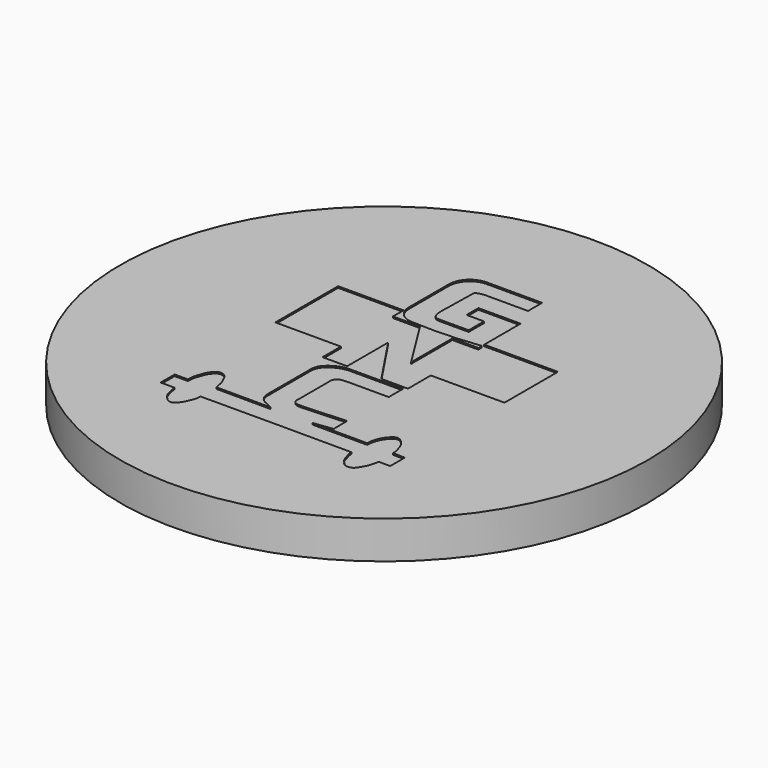
from build123d import *

# Parameters (mm, degrees)
F0_R     = 44.45
F1_DEPTH = 6.35
F3_DEPTH = 0.254


# Not quite as in the source:
# - ends of sketch curves that miss each other by under 0.0002 mm in the source are joined


with BuildPart() as f1:
    # F0 (on Top) → F1 (new body)
    with BuildSketch(Plane.XY):
        Circle(F0_R)
    extrude(amount=F1_DEPTH)

    # F2 (on face) → F3 (cut)
    with BuildSketch(Plane.XY.offset(6.35)):
        with BuildLine():
            Line((5.6039993651, 23.2917912652), (5.6039993651, 26.2641511811))
            Line((5.6039993651, 26.2641511811), (-3.5374157604, 26.2641511811))
            ThreePointArc((-3.5374157604, 26.2641511811), (-6.1724008767, 25.2877017598), (-7.2804156008, 22.7052797559))
            Line((-7.2804156008, 22.7052797559), (-7.2804156008, 14.3152289093))
            ThreePointArc((-7.2804156008, 14.3152289093), (-6.4557803762, 12.2478717336), (-4.4346582144, 11.3156409934))
            ThreePointArc((-4.4346582144, 11.3156409934), (1.3092272973, 11.2673019991), (7.0349466987, 11.7263169959))
            Line((7.0349466987, 11.7263169959), (7.0961336605, 12.2146336362))
            Line((7.0961336605, 12.2146336362), (7.0961336605, 19.8627323627))
            Line((7.0961336605, 19.8627323627), (0, 19.8627323627))
            Line((0, 19.8627323627), (0, 17.358450219))
            Line((0, 17.358450219), (2.9400843196, 17.3616167158))
            Line((2.9400843196, 17.3616167158), (2.9400843196, 14.1317071393))
            Line((2.9400843196, 14.1317071393), (0, 14.1317071393))
            Line((0, 14.1317071393), (-2.2346060723, 14.1317071393))
            ThreePointArc((-2.2346060723, 14.1317071393), (-2.7898678793, 14.3800667532), (-3.1146267429, 14.8943914101))
            ThreePointArc((-3.1146267429, 14.8943914101), (-3.2355914853, 15.5005322545), (-3.2674165577, 16.1178055789))
            Line((-3.2674165577, 16.1178055789), (-3.1592417437, 21.2145812126))
            ThreePointArc((-3.1592417437, 21.2145812126), (-3.1837866635, 21.575252567), (-3.1439608429, 21.9345577061))
            ThreePointArc((-3.1439608429, 21.9345577061), (-3.117530452, 22.198564373), (-3.1439608429, 22.4625710398))
            ThreePointArc((-3.1439608429, 22.4625710398), (-3.0817290753, 22.8241742068), (-2.7919525746, 23.0492502451))
            ThreePointArc((-2.7919525746, 23.0492502451), (-2.1422008965, 23.2306538656), (-1.4703774561, 23.2917912652))
            Line((-1.4703774561, 23.2917912652), (5.6039993651, 23.2917912652))
        make_face()
        with BuildLine():
            Line((-3.1592417437, 21.2145812126), (-3.1439608429, 21.9345577061))
            ThreePointArc((-3.1439608429, 21.9345577061), (-3.1837866635, 21.575252567), (-3.1592417437, 21.2145812126))
        make_face()
        Polygon((7.0961336605, 12.2146336362), (7.0349466987, 11.7263169959), (7.0961336605, 10.9925279394), (7.0961336605, 0.9659290663), (19.5016358048, 0.9659290663), (19.5016358048, 12.2146336362), align=None)
        Polygon((7.0961336605, 0.9659290663), (7.0961336605, 10.9925279394), (2.7143813204, 10.9925279394), (2.7143813204, 2.2997791572), (-2.7398910557, 10.9925279394), (-7.300500758, 10.9925279394), (-7.2804156008, 0), (-7.2804156008, -3.8537723012), (-6.2781353481, -3.8537723012), (-3.1410043308, -3.8537723012), (-3.1410043308, 4.7863919603), (2.6191033489, -3.8537723012), (7.0961336605, -3.8537723012), align=None)
        Polygon((-7.2804156008, 0), (-7.300500758, 10.9925279394), (-7.2804156008, 13.206558302), (-18.3086954057, 13.206558302), (-18.3086954057, 0), align=None)
        with BuildLine():
            Line((0, -7.2983574902), (6.6179535352, -7.2983574902))
            Line((6.6179535352, -7.2983574902), (6.6179535352, -4.2878086955))
            Line((6.6179535352, -4.2878086955), (-2.2489061664, -4.2878086955))
            ThreePointArc((-2.2489061664, -4.2878086955), (-4.0568875501, -4.6442817118), (-5.5942512015, -5.6603440615))
            ThreePointArc((-5.5942512015, -5.6603440615), (-6.1507192567, -6.4794007942), (-6.3533238135, -7.4486592847))
            Line((-6.3533238135, -7.4486592847), (-6.3533238135, -16.6105034737))
            ThreePointArc((-6.3533238135, -16.6105034737), (-5.8759308245, -17.9913268961), (-4.6476325952, -18.782440573))
            Line((-4.6476325952, -18.782440573), (-3.7075637703, -19.2863568686))
            Line((-3.7075637703, -19.2863568686), (3.3881619917, -19.303988614))
            Line((3.3881619917, -19.303988614), (6.6293859856, -18.9052186906))
            Line((6.6293859856, -18.9052186906), (6.593650474, -16.0276701207))
            Line((6.593650474, -16.0276701207), (0, -16.3928680122))
            ThreePointArc((0, -16.3928680122), (-0.7145080017, -16.4126398372), (-1.4290160034, -16.3928680122))
            ThreePointArc((-1.4290160034, -16.3928680122), (-2.080113152, -16.0523673946), (-2.251843689, -15.3379607946))
            Line((-2.251843689, -15.3379607946), (-2.251843689, -8.4599647671))
            ThreePointArc((-2.251843689, -8.4599647671), (-2.0899663646, -7.8730095416), (-1.6501033679, -7.4520092458))
            ThreePointArc((-1.6501033679, -7.4520092458), (-0.8286208401, -7.3368533365), (0, -7.2983574902))
        make_face()
        with BuildLine():
            Line((3.3881619917, -19.303988614), (-3.7075637703, -19.2863568686))
            Line((-3.7075637703, -19.2863568686), (-12.6563319936, -19.2641206086))
            Line((-12.6563319936, -19.2641206086), (-12.8377182409, -19.2641206086))
            Line((-12.8377182409, -19.2641206086), (-12.9873463884, -18.6591409147))
            ThreePointArc((-12.9873463884, -18.6591409147), (-13.1098010784, -17.8878071535), (-13.4031539783, -17.1640012413))
            ThreePointArc((-13.4031539783, -17.1640012413), (-13.5725884432, -16.8395453931), (-13.7304924428, -16.5093243122))
            ThreePointArc((-13.7304924428, -16.5093243122), (-14.0521811274, -16.0543913958), (-14.5178735256, -15.7484859228))
            ThreePointArc((-14.5178735256, -15.7484859228), (-15.086809482, -15.6747136098), (-15.6148988754, -15.8988833427))
            ThreePointArc((-15.6148988754, -15.8988833427), (-16.1466107031, -16.4449553577), (-16.5172908455, -17.1109195799))
            ThreePointArc((-16.5172908455, -17.1109195799), (-16.7501696159, -17.7330376736), (-16.9609729201, -18.3629784733))
            ThreePointArc((-16.9609729201, -18.3629784733), (-17.0934179213, -18.9312665088), (-17.1379111707, -19.5130854845))
            Line((-17.1379111707, -19.5130854845), (-17.1379111707, -19.8522191495))
            Line((-17.1379111707, -19.8522191495), (-19.3871874362, -19.8522191495))
            Line((-19.3871874362, -19.8522191495), (-19.3871874362, -22.8021256626))
            Line((-19.3871874362, -22.8021256626), (-17.0194374538, -22.8021256626))
            Line((-17.0194374538, -22.8021256626), (-17.0194374538, -23.2551640704))
            ThreePointArc((-17.0194374538, -23.2551640704), (-16.9093551317, -23.6838787474), (-16.7950224131, -24.1114795208))
            ThreePointArc((-16.7950224131, -24.1114795208), (-16.7338426372, -24.3328635786), (-16.6711639613, -24.5538279414))
            ThreePointArc((-16.6711639613, -24.5538279414), (-16.4738073507, -25.0326716474), (-16.1757338792, -25.4562199116))
            ThreePointArc((-16.1757338792, -25.4562199116), (-15.9267297619, -25.732701627), (-15.6729177634, -26.0047763574))
            ThreePointArc((-15.6729177634, -26.0047763574), (-14.9718242273, -26.3117655956), (-14.2623546636, -26.0246637372))
            ThreePointArc((-14.2623546636, -26.0246637372), (-13.7772653209, -25.4368959002), (-13.4154763073, -24.7661564499))
            ThreePointArc((-13.4154763073, -24.7661564499), (-13.2751868701, -24.4473909933), (-13.1237693131, -24.1337586194))
            ThreePointArc((-13.1237693131, -24.1337586194), (-12.9090296801, -23.5454392253), (-12.837051295, -22.9233042467))
            Line((-12.837051295, -22.9233042467), (-12.8377182409, -22.622095421))
            Line((-12.8377182409, -22.622095421), (0.5678676759, -22.592412358))
            Line((0.5678676759, -22.592412358), (12.5019904939, -22.6220667474))
            Line((12.5019904939, -22.6220667474), (12.5135298725, -22.622095421))
            Line((12.5135298725, -22.622095421), (12.6259239413, -22.622095421))
            Line((12.6259239413, -22.622095421), (12.6259239413, -22.8433404118))
            ThreePointArc((12.6259239413, -22.8433404118), (12.6900931034, -23.3765945805), (12.878936831, -23.8794024329))
            ThreePointArc((12.878936831, -23.8794024329), (13.1121897024, -24.7032143779), (13.6001783309, -25.4067341867))
            Line((13.6001783309, -25.4067341867), (13.7601625174, -25.5711600184))
            ThreePointArc((13.7601625174, -25.5711600184), (14.0077931702, -25.8774350672), (14.3499616533, -26.0724890977))
            ThreePointArc((14.3499616533, -26.0724890977), (14.8915415981, -26.1493664388), (15.4228175364, -26.0191172952))
            ThreePointArc((15.4228175364, -26.0191172952), (15.5930961418, -25.9161088082), (15.7359875739, -25.7775895298))
            ThreePointArc((15.7359875739, -25.7775895298), (16.5550328697, -24.4671777543), (17.0114282519, -22.9907911271))
            Line((17.0114282519, -22.9907911271), (17.0942133791, -22.5096959621))
            Line((17.0942133791, -22.5096959621), (19.0433021635, -22.5096959621))
            Line((19.0433021635, -22.5096959621), (19.0433021635, -19.4356404245))
            Line((19.0433021635, -19.4356404245), (17.0150939375, -19.4110530503))
            Line((17.0150939375, -19.4110530503), (17.0150939375, -19.0368138024))
            ThreePointArc((17.0150939375, -19.0368138024), (16.989674065, -18.7347053505), (16.9141292572, -18.4410922229))
            Line((16.9141292572, -18.4410922229), (16.690004617, -17.6846757531))
            ThreePointArc((16.690004617, -17.6846757531), (16.407642716, -17.0034564681), (15.9896202385, -16.3959655911))
            ThreePointArc((15.9896202385, -16.3959655911), (15.6603689447, -16.0642729564), (15.2857392253, -15.7848467735))
            ThreePointArc((15.2857392253, -15.7848467735), (14.6670179234, -15.6398096454), (14.0927875351, -15.9120435136))
            Line((14.0927875351, -15.9120435136), (13.9366754533, -16.0662262266))
            ThreePointArc((13.9366754533, -16.0662262266), (13.2239743808, -16.988100564), (12.7797400013, -18.0653428434))
            ThreePointArc((12.7797400013, -18.0653428434), (12.7644443964, -18.1246889663), (12.7497899169, -18.1841966471))
            ThreePointArc((12.7497899169, -18.1841966471), (12.6499744154, -18.7132948986), (12.6030528918, -19.2496776581))
            Line((12.6030528918, -19.2496776581), (12.6030528918, -19.3145554513))
            Line((12.6030528918, -19.3145554513), (9.0023325756, -19.3145554513))
            Line((9.0023325756, -19.3145554513), (3.3881619917, -19.303988614))
        make_face()
    extrude(amount=-F3_DEPTH, mode=Mode.SUBTRACT)


solid = f1.part
